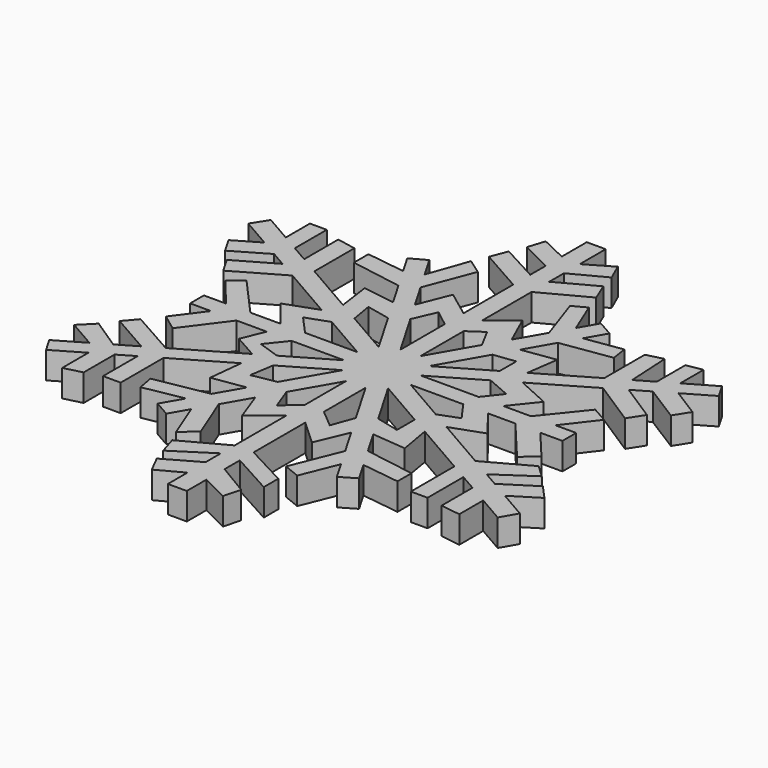
from build123d import *

# Parameters (mm, degrees)
F1_DEPTH = 5.08


# Not quite as in the source:
# - a feature names something its author has since deleted; it is built from what else it names


with BuildPart() as f1:
    # F0 (on Top) → F1 (new body)
    with BuildSketch(Plane.XY):
        Polygon((-15.1521363896, 6.8187847033), (-6.1961833334, 1.6591490712), (-2.8812128358, 1.6591490712), (-4.76298338, 4.8910336511), (-13.2476550799, 9.7791582487), (-17.2520195764, 12.0861222994), (-27.2555859428, 17.8493009526), (-30.8494522007, 19.9197718767), (-34.1122900736, 21.7995332427), (-37.2971609959, 23.6343768815), (-42.5028508198, 26.6334393527), (-44.3895836961, 23.6628407147), (-38.7390896331, 20.4075210046), (-35.3380082744, 18.4481158518), (-32.418172927, 16.7659624949), (-28.9448541734, 14.764940483), (-18.7254680578, 8.8774253957), align=None)
        Polygon((-37.2971609959, 23.6343768815), (-34.1122900736, 21.7995332427), (-34.1122900736, 29.3374934699), (-37.2971609959, 29.3374934699), align=None)
        Polygon((-41.6546580982, 14.7670020815), (-35.3380082744, 18.4481158518), (-38.7390896331, 20.4075210046), (-43.3692743738, 17.7092177452), align=None)
        Polygon((-37.8834722233, 9.6244753804), (-28.9448541734, 14.764940483), (-32.418172927, 16.7659624949), (-39.6114529464, 12.6292151021), align=None)
        Polygon((-30.8494522007, 19.9197718767), (-27.2555859428, 17.8493009526), (-27.2555859428, 27.2804812994), (-30.8494522007, 27.9661507811), align=None)
        Polygon((-24.4486728352, 23.661946645), (-14.7335412409, 22.0151683141), (-17.0989244778, 26.0776432169), (-24.4486728352, 27.0902977791), align=None)
        Polygon((-13.9303403776, 27.1979285617), (-11.8319710741, 23.5940420966), (-8.3354241815, 32.7470765915), (-11.2495222729, 34.8040850367), align=None)
        Polygon((-9.4712365479, 12.9773175279), (-4.76298338, 4.8910336511), (-1.7208857771, 3.1384434924), (-1.7208857771, 6.2285557687), (-6.6895745189, 14.7621299477), (-9.0301347199, 18.7819720297), (-11.8319710741, 23.5940420966), (-13.9303403776, 27.1979285617), (-16.2757938397, 31.2261746731), (-19.1711229872, 29.6365821268), (-17.0989244778, 26.0776432169), (-14.7335412409, 22.0151683141), (-12.0218611367, 17.3579389077), align=None)
        Polygon((-13.9495102358, 13.9542592224), (-9.4712365479, 12.9773175279), (-12.0218611367, 17.3579389077), (-18.1150609296, 18.2769985404), (-17.2520195764, 12.0861222994), (-13.2476550799, 9.7791582487), align=None)
        Polygon((-9.0301347199, 18.7819720297), (-6.6895745189, 14.7621299477), (-4.8024461739, 19.0735494252), (-1.7208857771, 16.6822017636), (-1.7208857771, 21.1120599415), (-6.637104847, 24.7813777532), align=None)
        Polygon((1.8570653028, 44.0727972891), (1.8570653028, 40.3380580246), (8.1761362362, 43.6650940683), (6.7491796199, 46.9267086592), align=None)
        Polygon((1.8570653028, 36.8542575743), (1.8570653028, 32.6936468482), (10.4184974316, 37.2437888291), (8.9915398839, 40.7092550304), align=None)
        Polygon((9.0497794959, 32.759775339), (12.0121748618, 24.1092241589), (14.1400860829, 27.8027936982), (11.5600488333, 34.0939074939), align=None)
        Polygon((16.9943218466, 25.851042646), (15.0253487413, 22.4333534993), (24.4589996778, 23.859241042), (23.9979358721, 26.9096323755), align=None)
        Polygon((6.7068845063, 14.9004476559), (1.8570653028, 6.4822654015), (1.8570653028, 3.0360630773), (4.8564502526, 4.7824602983), (9.8637657614, 13.4740202905), (12.0351058955, 17.2429725378), (15.0253487413, 22.4333534993), (16.9943218466, 25.851042646), (19.1071601501, 29.5184490309), (16.1199634229, 31.2394101142), (14.1400860829, 27.8027936982), (12.0121748618, 24.1092241589), (9.0660807462, 18.9954753443), align=None)
        Polygon((12.0351058955, 17.2429725378), (9.8637657614, 13.4740202905), (13.9518412161, 13.9772777911), (13.9518412161, 10.078267862), (17.4944029143, 12.1409307108), (18.334635939, 18.1562227663), align=None)
        Polygon((4.8564502526, 4.7824602983), (3.0570719177, 1.6591490712), (5.7764827992, 1.6591490712), (14.7676641447, 6.8942803994), (18.8851145535, 9.2916732224), (29.2332933727, 15.3169187429), (32.5454687799, 17.2454387641), (35.6516697131, 19.0540297815), (38.9510449864, 20.9750969019), (44.1476161695, 24.0008097148), (42.5565533967, 26.7334123995), (37.1827887702, 23.604528389), (34.1619707935, 21.8456517499), (30.9930839806, 20.0005617676), (27.4081488881, 17.9132269345), (17.4944029143, 12.1409307108), (13.9518412161, 10.078267862), align=None)
        Polygon((27.4081488881, 27.4701060262), (27.4081488881, 17.9132269345), (30.9930839806, 20.0005617676), (30.5355446744, 28.2631905284), align=None)
        Polygon((34.1619707935, 28.6073924508), (34.1619707935, 21.8456517499), (37.1827887702, 23.604528389), (37.1827887702, 29.1170196142), align=None)
        Polygon((38.9510449864, 20.9750969019), (35.6516697131, 19.0540297815), (42.5163951244, 14.7359767381), (44.3175727833, 17.5994408783), align=None)
        Polygon((32.5454687799, 17.2454387641), (29.2332933727, 15.3169187429), (37.8070259376, 9.7949526326), (39.6560350764, 12.665834045), align=None)
        Polygon((19.2876899946, 4.9391330685), (16.6940460313, 1.6591490712), (21.3311681855, 1.6591490712), (25.1636425364, 6.4347924199), (18.8851145535, 9.2916732224), (14.7676641447, 6.8942803994), align=None)
        Polygon((3.3247213854, 0.2316066278), (6.4815483453, -1.5870805364), (16.3882686156, -1.5870805364), (21.0253907699, -1.5870805364), (26.2311057705, -1.5870805364), (30.9320869255, -1.5870805364), (35.1013163436, -1.5870805364), (35.1013163436, 1.6591490712), (31.1964484263, 1.6591490712), (26.5701165754, 1.6591490712), (21.3311681855, 1.6591490712), (16.6940460313, 1.6591490712), (5.7764827992, 1.6591490712), align=None)
        Polygon((32.6504404056, 9.2291308101), (26.5701165754, 1.6591490712), (31.1964484263, 1.6591490712), (35.6906051147, 7.51077733), align=None)
        Polygon((30.9320869255, -1.5870805364), (26.2311057705, -1.5870805364), (33.0601913193, -9.7397571839), (35.8227821398, -7.4256743537), align=None)
        Polygon((21.0253907699, -1.5870805364), (16.3882686156, -1.5870805364), (18.981912579, -5.2229894791), (15.2440576262, -6.6352708104), (18.9944182437, -8.7959000761), (25.0337509769, -6.6377045587), align=None)
        Polygon((6.4815483453, -1.5870805364), (2.8297823608, -1.5870805364), (4.5415518059, -4.5269933176), (13.873220827, -9.9030835769), (17.4029516402, -11.9366052759), (27.759747054, -17.9032835642), (30.9267255698, -19.7278191657), (34.104432385, -21.5585354735), (37.8597208497, -23.7220037331), (42.9251531775, -26.6402621213), (44.6802444637, -23.5938231305), (39.4184178153, -20.5624195384), (35.8812669625, -18.5246230625), (33.0539132507, -16.8957495228), (29.1046865765, -14.6205510554), (18.9944182437, -8.7959000761), (15.2440576262, -6.6352708104), align=None)
        Polygon((37.4089548695, -10.0692948326), (29.1046865765, -14.6205510554), (33.0539132507, -16.8957495228), (39.7882158268, -12.3163715471), align=None)
        Polygon((41.903111558, -14.6956292447), (35.8812669625, -18.5246230625), (39.4184178153, -20.5624195384), (44.4145495403, -17.4714301247), align=None)
        Polygon((37.8597208497, -23.7220037331), (34.104432385, -21.5585354735), (34.104432385, -28.8389942143), (37.8597208497, -29.3677190784), align=None)
        Polygon((30.9267255698, -19.7278191657), (27.759747054, -17.9032835642), (27.759747054, -28.1780904625), (30.9267255698, -28.1780904625), align=None)
        Polygon((13.873220827, -14.1042571049), (9.4815203496, -13.0112414161), (12.0122463527, -17.3576875705), (18.4317468065, -17.9554254282), (17.4029516402, -11.9366052759), (13.873220827, -9.9030835769), align=None)
        Polygon((24.1908593434, -23.5517548863), (14.7232563734, -22.0137661285), (16.9830221391, -25.8948461863), (24.1908593434, -26.8562792335), align=None)
        Polygon((14.2648872791, -27.7887646172), (12.1212640639, -24.1071559133), (8.3815095316, -33.3992776126), (11.5014840248, -34.6549584065), align=None)
        Polygon((1.8570653028, -2.9804273487), (1.8570653028, -6.4787017943), (6.7604426255, -14.900105566), (9.1345656921, -18.9775908649), (12.1212640639, -24.1071559133), (14.2648872791, -27.7887646172), (16.3153485402, -31.3103704538), (19.1688387153, -29.6489207247), (16.9830221391, -25.8948461863), (14.7232563734, -22.0137661285), (12.0122463527, -17.3576875705), (9.4815203496, -13.0112414161), (4.5415518059, -4.5269933176), align=None)
        Polygon((9.1345656921, -18.9775908649), (6.7604426255, -14.900105566), (5.2277389314, -19.1343550105), (1.8570653028, -16.3049248513), (1.8570653028, -20.7062608097), (6.5638585347, -25.0290019903), align=None)
        Polygon((9.9420179013, -37.1725151781), (1.8570653028, -32.8870771918), (1.8570653028, -36.1440090928), (9.9420179013, -40.6008644495), align=None)
        Polygon((7.885006662, -43.3435461018), (1.8570653028, -39.7437775973), (1.8570653028, -44.0292155836), (7.0279198098, -46.6004780028), align=None)
        Polygon((-8.3996593621, -32.544236863), (-11.7709384883, -24.0789019429), (-13.9461838751, -27.8546328198), (-11.1423391518, -34.9440837745), align=None)
        Polygon((-16.675518786, -25.6860823162), (-14.6477497461, -22.1663368099), (-24.7280347434, -24.0127665043), (-24.1700714123, -27.0588772837), align=None)
        Polygon((-11.8567255223, -17.3217540313), (-9.4281872071, -13.1063642834), (-13.9495102358, -13.9470666181), (-13.230870294, -9.4079160698), (-17.3521867829, -11.8075599248), (-18.0364647549, -18.2698073331), align=None)
        Polygon((-6.1961833334, 1.6591490712), (-3.3368888311, 0.0118740459), (-2.2802893501, 0.6270809728), (-2.8812128358, 1.6591490712), align=None)
        Polygon((-0.4809075611, 2.4240766632), (-0.9215918339, 1.6591490712), (-0.5077432854, 1.6591490712), (0.1659550199, 2.0514111076), align=None)
        Polygon((0.0041014299, 3.2659418771), (-0.4809075611, 2.4240766632), (0.1659550199, 2.0514111076), (0.573200825, 2.2885307018), align=None)
        Polygon((0.1659550199, 2.0514111076), (-0.5077432854, 1.6591490712), (0.8468326311, 1.6591490712), align=None)
        Polygon((2.5062891661, 0.7031155799), (2.0039768431, -0.1687842799), (2.1642635977, -0.4440719828), (3.3247213854, 0.2316066278), align=None)
        Polygon((3.0570719177, 1.6591490712), (2.5062891661, 0.7031155799), (3.3247213854, 0.2316066278), (5.7764827992, 1.6591490712), align=None)
        Polygon((2.1642635977, -0.4440719828), (2.8297823608, -1.5870805364), (6.4815483453, -1.5870805364), (3.3247213854, 0.2316066278), align=None)
        Polygon((-2.7917849723, -1.5870805364), (-6.0830454624, -1.5870805364), (-14.7410023167, -6.628191312), (-17.9388041921, -8.4901171409), (-29.0659878789, -14.968939631), (-32.213328117, -16.8014840819), (-35.8265301636, -18.9052773991), (-38.8972862931, -20.6932306165), (-44.0705799466, -23.7053900464), (-42.4795171739, -26.4379927311), (-37.0263872337, -23.2628981256), (-33.6568966786, -21.3010062576), (-30.6839389395, -19.569996327), (-27.3549464236, -17.6316845144), (-17.3521867829, -11.8075599248), (-13.230870294, -9.4079160698), (-4.3025161437, -4.2093659877), align=None)
        Polygon((-0.1781224656, -1.8079304339), (-0.6892265774, -2.1055217119), (0.1036661127, -3.4672911722), (0.75119788, -2.3433234109), align=None)
        Polygon((1.1868787793, -1.5870805364), (0.2011806222, -1.5870805364), (-0.1781224656, -1.8079304339), (0.75119788, -2.3433234109), align=None)
        Polygon((1.684420393, -0.7234615421), (0.2011806222, -1.5870805364), (1.1868787793, -1.5870805364), align=None)
        Polygon((-0.5614676193, -1.5870805364), (-0.9910898738, -1.5870805364), (-0.6892265774, -2.1055217119), (-0.1781224656, -1.8079304339), align=None)
        Polygon((-1.2079462696, -1.214636168), (-0.9910898738, -1.5870805364), (-0.5614676193, -1.5870805364), align=None)
        Polygon((0.2011806222, -1.5870805364), (-0.5614676193, -1.5870805364), (-0.1781224656, -1.8079304339), align=None)
        Polygon((0.1659550199, 2.0514111076), (0.8468326311, 1.6591490712), (0.9396593987, 1.6591490712), (0.573200825, 2.2885307018), align=None)
        Polygon((-0.9215918339, 1.6591490712), (-1.1304862841, 1.2965558528), (-0.5077432854, 1.6591490712), align=None)
        Polygon((0.9396593987, 1.6591490712), (0.8468326311, 1.6591490712), (0.9865146955, 1.5786765015), align=None)
        Polygon((-3.3368888311, 0.0118740459), (-6.0830454624, -1.5870805364), (-2.7917849723, -1.5870805364), (-2.2359988472, -0.6223623276), align=None)
        Polygon((-1.7208857771, -2.7062071156), (-4.3025161437, -4.2093659877), (-9.4281872071, -13.1063642834), (-11.8567255223, -17.3217540313), (-14.6477497461, -22.1663368099), (-16.675518786, -25.6860823162), (-18.9087183617, -29.562408474), (-15.9215216345, -31.2833695573), (-13.9461838751, -27.8546328198), (-11.7709384883, -24.0789019429), (-8.8876021743, -19.0740863872), (-6.4250674811, -14.7996866652), (-1.7208857771, -6.6342979608), align=None)
        Polygon((-27.3549464236, -27.7445467655), (-27.3549464236, -17.6316845144), (-30.6839389395, -19.569996327), (-30.6839389395, -27.7445467655), align=None)
        Polygon((-33.6568966786, -28.6016336177), (-33.6568966786, -21.3010062576), (-37.0263872337, -23.2628981256), (-37.0263872337, -29.4587223325), align=None)
        Polygon((-38.8972862931, -20.6932306165), (-35.8265301636, -18.9052773991), (-41.6546580982, -15.0596497115), (-44.2259205174, -17.6309125964), align=None)
        Polygon((-32.213328117, -16.8014840819), (-29.0659878789, -14.968939631), (-37.7120567155, -10.0885411957), (-39.7690651607, -12.4883865938), align=None)
        Polygon((-26.3984990906, -1.5870805364), (-31.2329256963, -1.5870805364), (-35.3335314167, -7.0861193969), (-32.2266952735, -9.4028715394), align=None)
        Polygon((-35.1700005722, 1.6591490712), (-35.1700005722, -1.5870805364), (-31.2329256963, -1.5870805364), (-26.3984990906, -1.5870805364), (-20.708704893, -1.5870805364), (-15.992986564, -1.5870805364), (-6.0830454624, -1.5870805364), (-3.3368888311, 0.0118740459), (-6.1961833334, 1.6591490712), (-16.0715827387, 1.6591490712), (-20.708704893, 1.6591490712), (-26.3984990906, 1.6591490712), (-31.0267718178, 1.6591490712), align=None)
        Polygon((-35.6550445449, 7.3960458394), (-31.0267718178, 1.6591490712), (-26.3984990906, 1.6591490712), (-33.2598102906, 9.3284141253), align=None)
        Polygon((-24.7170651, 6.7234931048), (-20.708704893, 1.6591490712), (-16.0715827387, 1.6591490712), (-19.3725848239, 5.3087777924), (-15.1521363896, 6.8187847033), (-18.7254680578, 8.8774253957), align=None)
        Polygon((-1.7208857771, 16.6822017636), (-1.7208857771, 6.2285557687), (0.0041014299, 3.2659418771), (1.8570653028, 6.4822654015), (1.8570653028, 16.6822017636), (1.8570653028, 21.1120599415), (1.8570653028, 32.6936468482), (1.8570653028, 36.8542575743), (1.8570653028, 40.3380580246), (1.8570653028, 44.0727972891), (1.8570653028, 50.182213774), (-1.7208857771, 50.182213774), (-1.7208857771, 44.2882649159), (-1.7208857771, 40.4905730393), (-1.7208857771, 36.8542575743), (-1.7208857771, 32.8279853171), (-1.7208857771, 21.1120599415), align=None)
        Polygon((-7.6223118831, 43.4612424579), (-1.7208857771, 40.4905730393), (-1.7208857771, 44.2882649159), (-6.6030570906, 46.6209331062), align=None)
        Polygon((-10.0685232919, 37.5495643821), (-1.7208857771, 32.8279853171), (-1.7208857771, 36.8542575743), (-8.8454178203, 40.7092550304), align=None)
        Polygon((-4.8324564141, -19.0557606984), (-6.4250674811, -14.7996866652), (-8.8876021743, -19.0740863872), (-6.7973384303, -24.7932171915), (-1.7208857771, -20.7062608097), (-1.7208857771, -16.3049248513), align=None)
        Polygon((-1.7208857771, -36.1440090928), (-1.7208857771, -32.8870771918), (-9.9424166274, -37.3439306859), (-8.9139119391, -40.7722799573), align=None)
        Polygon((0.1036661127, -3.4672911722), (-1.7208857771, -6.6342979608), (-1.7208857771, -16.3049248513), (-1.7208857771, -20.7062608097), (-1.7208857771, -32.8870771918), (-1.7208857771, -36.1440090928), (-1.7208857771, -39.7437775973), (-1.7208857771, -44.0292155836), (-1.7208857771, -48.6534482334), (1.8570653028, -48.6534482334), (1.8570653028, -44.0292155836), (1.8570653028, -39.7437775973), (1.8570653028, -36.1440090928), (1.8570653028, -32.8870771918), (1.8570653028, -20.7062608097), (1.8570653028, -16.3049248513), (1.8570653028, -6.4787017943), align=None)
        Polygon((1.8570653028, 6.4822654015), (0.0041014299, 3.2659418771), (0.573200825, 2.2885307018), (1.8570653028, 3.0360630773), align=None)
        Polygon((-1.7208857771, 6.2285557687), (-1.7208857771, 3.1384434924), (-0.4809075611, 2.4240766632), (0.0041014299, 3.2659418771), align=None)
        Polygon((-4.76298338, 4.8910336511), (-2.8812128358, 1.6591490712), (-1.7208857771, 1.6591490712), (-1.7208857771, 3.1384434924), align=None)
        Polygon((-2.2802893501, 0.6270809728), (-3.3368888311, 0.0118740459), (-2.2359988472, -0.6223623276), (-1.8962093005, -0.0325650152), align=None)
        Polygon((-0.6892265774, -2.1055217119), (-1.7208857771, -2.7062071156), (-1.7208857771, -6.6342979608), (0.1036661127, -3.4672911722), align=None)
        Polygon((0.75119788, -2.3433234109), (0.1036661127, -3.4672911722), (1.8570653028, -6.4787017943), (1.8570653028, -2.9804273487), align=None)
        Polygon((2.8297823608, -1.5870805364), (1.8570653028, -1.5870805364), (1.8570653028, -2.9804273487), (4.5415518059, -4.5269933176), align=None)
        Polygon((1.8570653028, 3.0360630773), (1.8570653028, 1.6591490712), (3.0570719177, 1.6591490712), (4.8564502526, 4.7824602983), align=None)
        Polygon((0.573200825, 2.2885307018), (0.9396593987, 1.6591490712), (1.8570653028, 1.6591490712), (1.8570653028, 3.0360630773), align=None)
        Polygon((1.8570653028, 1.6591490712), (0.9396593987, 1.6591490712), (0.9865146955, 1.5786765015), (1.8570653028, 1.0771414996), align=None)
        Polygon((1.8570653028, 1.0771414996), (0.9865146955, 1.5786765015), (1.8570653028, 0.0835318929), align=None)
        Polygon((1.8570653028, 0.0835318929), (2.0039768431, -0.1687842799), (2.5062891661, 0.7031155799), (1.8570653028, 1.0771414996), align=None)
        Polygon((3.0570719177, 1.6591490712), (1.8570653028, 1.6591490712), (1.8570653028, 1.0771414996), (2.5062891661, 0.7031155799), align=None)
        Polygon((-1.2079462696, -1.214636168), (-0.5614676193, -1.5870805364), (0.2011806222, -1.5870805364), (1.684420393, -0.7234615421), (1.8570653028, -0.4237892749), (1.8570653028, 0.0835318929), (0.9865146955, 1.5786765015), (0.8468326311, 1.6591490712), (-0.5077432854, 1.6591490712), (-1.1304862841, 1.2965558528), (-1.7208857771, 0.2717567156), (-1.7208857771, -0.3336779184), align=None)
        Polygon((1.8570653028, 0.0835318929), (1.8570653028, -0.4237892749), (2.0039768431, -0.1687842799), align=None)
        Polygon((2.0039768431, -0.1687842799), (1.8570653028, -0.4237892749), (1.8570653028, -0.6229387363), (2.1642635977, -0.4440719828), align=None)
        Polygon((1.8570653028, -0.6229387363), (1.8570653028, -1.5870805364), (2.8297823608, -1.5870805364), (2.1642635977, -0.4440719828), align=None)
        Polygon((-1.7208857771, -1.5870805364), (-2.7917849723, -1.5870805364), (-4.3025161437, -4.2093659877), (-1.7208857771, -2.7062071156), align=None)
        Polygon((-1.7208857771, 3.1384434924), (-1.7208857771, 1.6591490712), (-0.9215918339, 1.6591490712), (-0.4809075611, 2.4240766632), align=None)
        Polygon((-2.8812128358, 1.6591490712), (-2.2802893501, 0.6270809728), (-1.7208857771, 0.952794698), (-1.7208857771, 1.6591490712), align=None)
        Polygon((-1.7208857771, 1.6591490712), (-1.7208857771, 0.952794698), (-1.1304862841, 1.2965558528), (-0.9215918339, 1.6591490712), align=None)
        Polygon((-1.7208857771, 0.952794698), (-2.2802893501, 0.6270809728), (-1.8962093005, -0.0325650152), (-1.7208857771, 0.2717567156), align=None)
        Polygon((-1.8962093005, -0.0325650152), (-2.2359988472, -0.6223623276), (-1.7208857771, -0.919125356), (-1.7208857771, -0.3336779184), align=None)
        Polygon((-2.2359988472, -0.6223623276), (-2.7917849723, -1.5870805364), (-1.7208857771, -1.5870805364), (-1.7208857771, -0.919125356), align=None)
        Polygon((-1.7208857771, -0.919125356), (-1.7208857771, -1.5870805364), (-0.9910898738, -1.5870805364), (-1.2079462696, -1.214636168), align=None)
        Polygon((-0.9910898738, -1.5870805364), (-1.7208857771, -1.5870805364), (-1.7208857771, -2.7062071156), (-0.6892265774, -2.1055217119), align=None)
        Polygon((1.8570653028, -1.5870805364), (1.1868787793, -1.5870805364), (0.75119788, -2.3433234109), (1.8570653028, -2.9804273487), align=None)
        Polygon((1.684420393, -0.7234615421), (1.1868787793, -1.5870805364), (1.8570653028, -1.5870805364), (1.8570653028, -0.6229387363), align=None)
        Polygon((1.8570653028, -0.4237892749), (1.684420393, -0.7234615421), (1.8570653028, -0.6229387363), align=None)
        Polygon((-1.1304862841, 1.2965558528), (-1.7208857771, 0.952794698), (-1.7208857771, 0.2717567156), align=None)
        Polygon((-1.7208857771, 0.2717567156), (-1.8962093005, -0.0325650152), (-1.7208857771, -0.3336779184), align=None)
        Polygon((-1.7208857771, -0.3336779184), (-1.7208857771, -0.919125356), (-1.2079462696, -1.214636168), align=None)
        Polygon((-15.992986564, -1.5870805364), (-20.708704893, -1.5870805364), (-22.4820952863, -5.9255908612), (-17.9388041921, -8.4901171409), (-14.7410023167, -6.628191312), (-18.9010133636, -5.2229904104), align=None)
        Polygon((4.7224564478, 18.6325535178), (6.7068845063, 14.9004476559), (9.0660807462, 18.9954753443), (6.5112816501, 24.6794500854), (1.8570653028, 21.1120599415), (1.8570653028, 16.6822017636), align=None)
        Polygon((-1.7208857771, -44.0292155836), (-1.7208857771, -39.7437775973), (-8.0568241556, -43.3435461018), (-6.4349750704, -46.5590826145), align=None)
    extrude(amount=F1_DEPTH)


solid = f1.part
